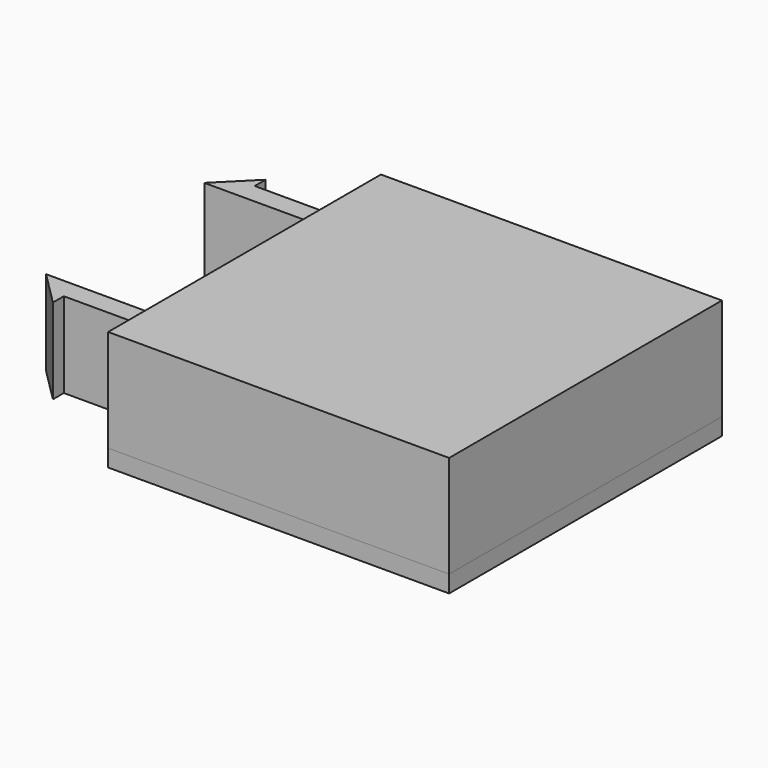
from build123d import *

# Parameters (mm, degrees)
F0_W     = 5
F0_H     = 1.2
F1_DEPTH = 5
F2_DEPTH = 1
F3_DEPTH = 6


with BuildPart() as f1:
    # F0 (on Top) → F1 (new body)
    with BuildSketch(Plane.XY):
        Polygon((-15, 5.8), (-15, 7), (-15, 7.8), (-17, 5.8), align=None)
        with Locations((-12.5, 6.4)):
            Rectangle(F0_W, F0_H)
    extrude(amount=F1_DEPTH)



with BuildPart() as f2:
    # F0 (on Top) → F2 (new body)
    with BuildSketch(Plane.XY):
        Polygon((10, -10), (10, 10), (-10, 10), (-10, 7), (-10, 5.8), (-10, -10), align=None)
    extrude(amount=-F2_DEPTH)


with BuildPart() as f1_1:
    add(f1.part)
    # F3 (add): a face of the model
    f3_faces = [f2.part.faces().sort_by_distance(p)[0] for p in [
        (0, 0, 0),
    ]]
    extrude(f3_faces, amount=F3_DEPTH)

    # F4: F1 across plane


with BuildPart() as f1_2:
    add(f1_1.part)
    add(f1_1.part.mirror(Plane.XZ))


solid = Compound([f2.part, f1_2.part])
